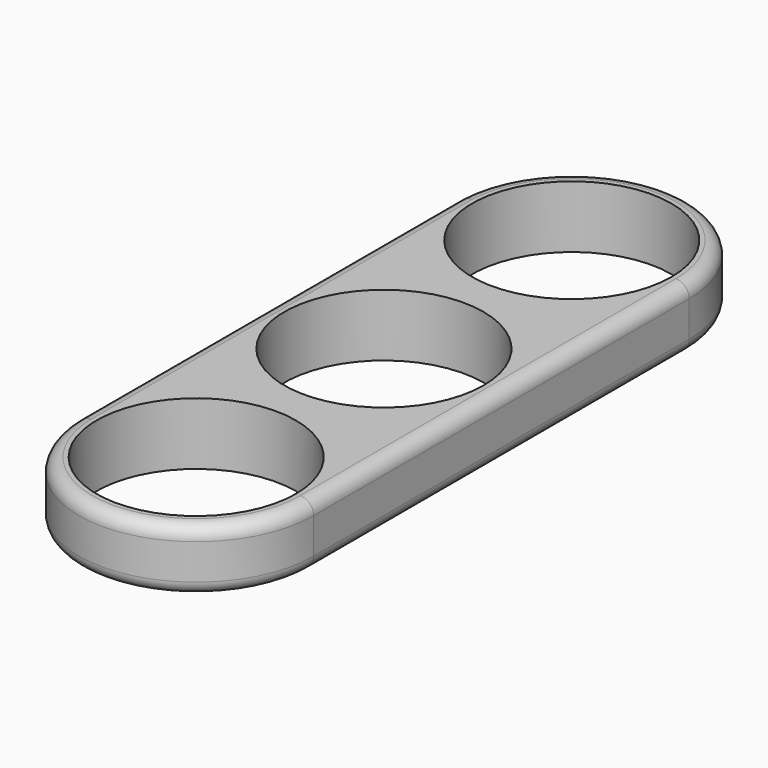
from build123d import *

# Parameters (mm, degrees)
F0_R     = 11.2
F1_DEPTH = 7
F2_R     = 1.5


with BuildPart() as f1:
    # F0 (on Top) → F1 (new body)
    with BuildSketch(Plane.XY):
        with BuildLine():
            Line((-13.1840748528, 25.7517945722), (-13.1840748528, 0.6482054278))
            Line((-13.1840748528, 0.6482054278), (-13.1840748528, -0.6482054278))
            Line((-13.1840748528, -0.6482054278), (-13.1840748528, -26.2634836304))
            Line((-13.1840748528, -26.2634836304), (-13.1840748528, -26.5365075959))
            ThreePointArc((-13.1840748528, -26.5365075959), (0.0853785885, -39.5998091598), (13.215218689, -26.3961906666))
            Line((13.215218689, -26.3961906666), (13.2, 26.4))
            ThreePointArc((13.2, 26.4), (0.3242005116, 39.5960181126), (-13.1840748528, 27.0482054278))
            Line((-13.1840748528, 27.0482054278), (-13.1840748528, 25.7517945722))
        make_face()
        Circle(F0_R, mode=Mode.SUBTRACT)
        with Locations((0.0152192374, -26.3999956132)):
            Circle(F0_R, mode=Mode.SUBTRACT)
        with Locations((0, 26.4)):
            Circle(F0_R, mode=Mode.SUBTRACT)
    extrude(amount=F1_DEPTH)

    # F2
    f2_edges = [f1.edges().sort_by_distance(p)[0] for p in [
        (0.085379, -39.599809, 0),
        (0.324201, 39.596018, 0),
        (0.324201, 39.596018, 7),
        (-13.184075, 0.255849, 7),
        (13.207609, 0.001905, 7),
        (13.207609, 0.001905, 0),
        (-13.184075, 0.255849, 0),
        (0.085379, -39.599809, 7),
    ]]
    fillet(f2_edges, radius=F2_R)


solid = f1.part
